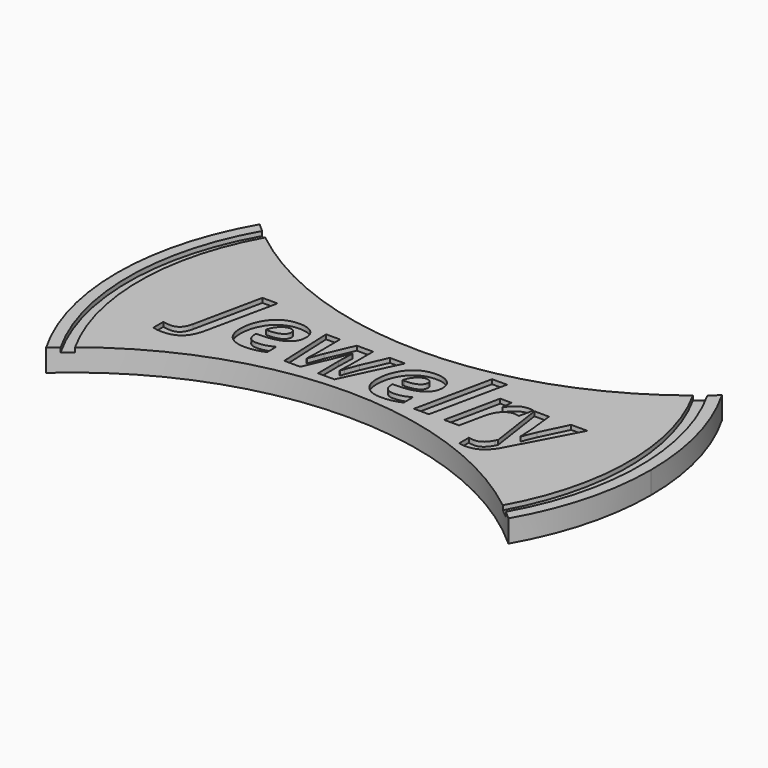
from build123d import *

# Parameters (mm, degrees)
F1_DEPTH     = 12.7
F2_TEXT_SIZE = 57.9782606413
F3_DEPTH     = 2.54
F5_DEPTH     = 2.54


# Not quite as in the source:
# - Text() gives the source's letters only with a copy of the font that has no kerning and outlines rounded to 1/6400 em; it was checked with that copy


with BuildPart() as f1:
    # F0 (on Top) → F1 (new body)
    with BuildSketch(Plane.XY):
        with BuildLine():
            ThreePointArc((131.9822715367, -76.2), (147.2070959265, -39.4440224736), (152.4, 0))
            ThreePointArc((152.4, 0), (147.2070959265, 39.4440224736), (131.9822715368, 76.2))
            ThreePointArc((131.9822715367, 76.2), (70.7106074079, 38.5384530031), (0, 25.4))
            ThreePointArc((0, 25.4), (-70.7106074079, 38.5384530031), (-131.9822715367, 76.2))
            ThreePointArc((-131.9822715368, 76.2), (-152.4, 0), (-131.9822715367, -76.2))
            ThreePointArc((-131.9822715367, -76.2), (0, -25.4), (131.9822715367, -76.2))
        make_face()
    extrude(amount=F1_DEPTH)

    # F2 (on face) → F3 (cut)
    with BuildSketch(Plane.XY.offset(12.7)):
        with Locations((-97.5774172693, -19.8285672814)):
            Text('Jewelry', F2_TEXT_SIZE, font='Open Sans', font_style=FontStyle.BOLDITALIC, text_align=(TextAlign.LEFT, TextAlign.BOTTOM))
    extrude(amount=-F3_DEPTH, mode=Mode.SUBTRACT)

    # F4 (on face) → F5 (cut)
    with BuildSketch(Plane.XY.offset(12.7)):
        with BuildLine():
            ThreePointArc((-122.1142413172, 67.8542922633), (-124.6264790463, 69.8749258556), (-127.1052869065, 71.9364326136))
            ThreePointArc((-127.1052869065, 71.9364326136), (-146.0500061512, 0), (-127.1052869065, -71.9364326136))
            ThreePointArc((-127.1052869065, -71.9364326136), (-124.6264790463, -69.8749258556), (-122.1142413172, -67.8542922633))
            ThreePointArc((-122.1142413172, -67.8542922633), (-139.7000104189, 0), (-122.1142413172, 67.8542922633))
        make_face()
        with BuildLine():
            ThreePointArc((127.1052821262, 71.9364285714), (124.6264707796, 69.8749190943), (122.1142294747, 67.8542828969))
            ThreePointArc((122.1142294747, 67.8542828969), (139.6999955177, 0), (122.1142294747, -67.8542828969))
            ThreePointArc((122.1142294747, -67.8542828969), (124.6264707796, -69.8749190943), (127.1052821262, -71.9364285714))
            ThreePointArc((127.1052821262, -71.9364285714), (146.05, 0), (127.1052821262, 71.9364285714))
        make_face()
    extrude(amount=-F5_DEPTH, mode=Mode.SUBTRACT)


solid = f1.part
